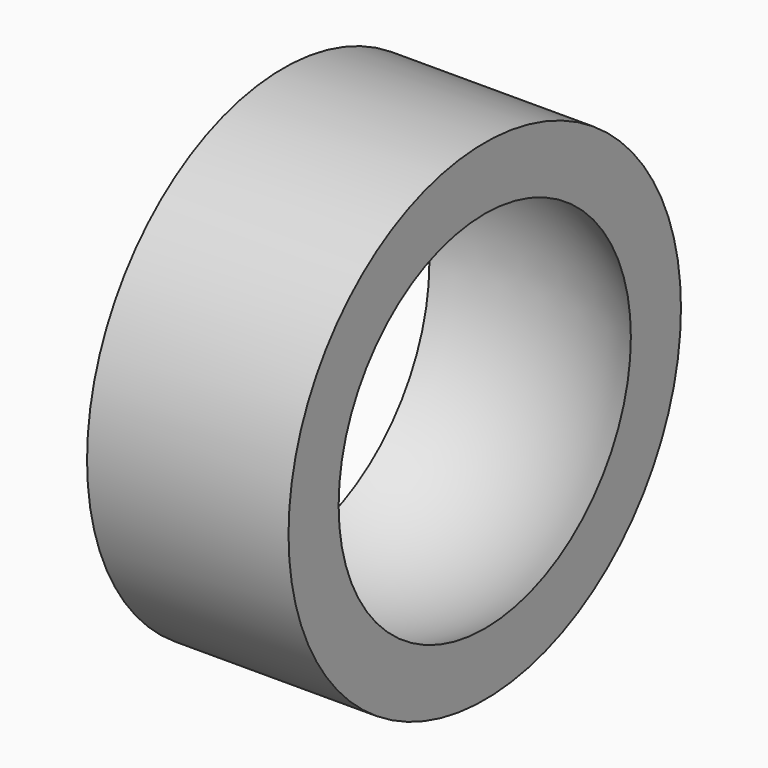
from build123d import *


# Not quite as in the source:
# - a feature names something its author has since deleted; it is built from what else it names


with BuildPart() as f1:
    # F0 (on Top) → F1 (revolve)
    with BuildSketch(Plane.XY):
        with BuildLine():
            ThreePointArc((-11.5, 20.8515024938), (0, 23.8125), (11.5, 20.8515024938))
            Line((11.5, 20.8515024938), (11.5, 28))
            Line((11.5, 28), (-11.5, 28))
            Line((-11.5, 28), (-11.5, 20.8515024938))
        make_face()
    revolve(axis=Axis((-0.2900734544, 0, 0), (1, 0, 0)))


solid = f1.part
